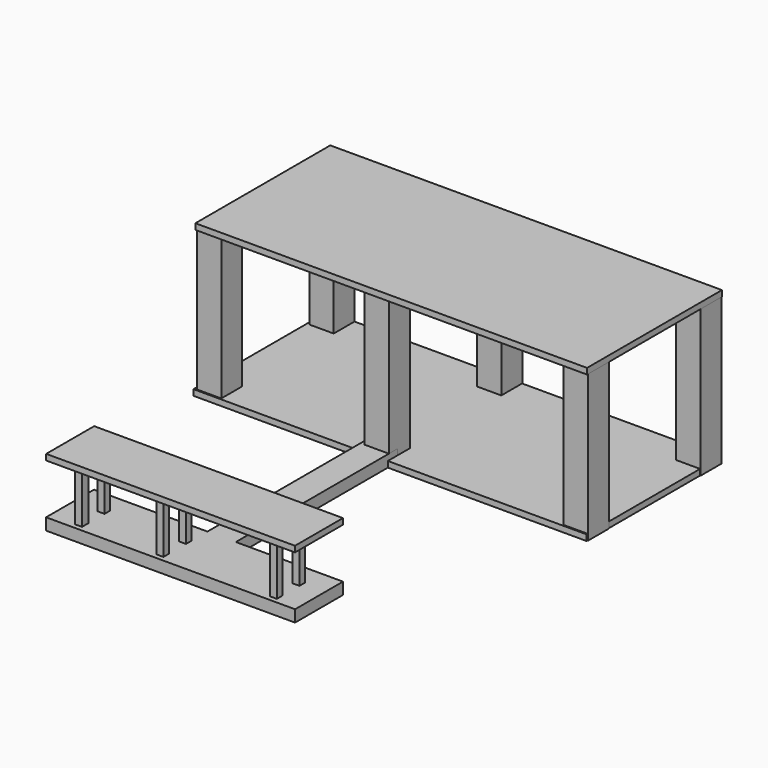
from build123d import *

# Parameters (mm, degrees)
F1_W      = 2.1082
F1_H      = 2.2606
F2_DEPTH  = 12.7
F0_W      = 2.4492868688
F0_H      = 17.4416182563
F3_DEPTH  = 1.016
F4_W      = 0.6096
F4_H      = 0.6012953818
F4_H_2    = 0.7112
F4_H_3    = 0.6096
F5_DEPTH  = 4.318
F6_W      = 21.482726559
F6_H      = 5.1775947213
F6_W_2    = 0.6096
F6_H_2    = 0.6012953818
F7_DEPTH  = 0.508
F8_W      = 33.9498203248
F8_H      = 14.4916079007
F9_DEPTH  = 0.508
F10_W     = 2.1082
F10_H     = 2.2606
F11_DEPTH = 0.508


# Not quite as in the source:
# - a feature names something its author has since deleted; it is built from what else it names


with BuildPart() as f2:
    # F1 (on Top) → F2 (new body)
    with BuildSketch(Plane.XY):
        with Locations((-15.5251261375, 6.3823008758)):
            Rectangle(F1_W, F1_H)
    extrude(amount=F2_DEPTH)


with BuildPart() as f2b:
    # F1 (on Top) → F2, piece 2 (new body)
    with BuildSketch(Plane.XY):
        with Locations((-15.5251261375, -5.7539824548)):
            Rectangle(F1_W, F1_H)
    extrude(amount=F2_DEPTH)


with BuildPart() as f2c:
    # F1 (on Top) → F2, piece 3 (new body)
    with BuildSketch(Plane.XY):
        with Locations((-1.0541, 6.3823008758)):
            Rectangle(F1_W, F1_H)
    extrude(amount=F2_DEPTH)


with BuildPart() as f2d:
    # F1 (on Top) → F2, piece 4 (new body)
    with BuildSketch(Plane.XY):
        with Locations((-1.0541, -5.7539824548)):
            Rectangle(F1_W, F1_H)
    extrude(amount=F2_DEPTH)


with BuildPart() as f2e:
    # F1 (on Top) → F2, piece 5 (new body)
    with BuildSketch(Plane.XY):
        with Locations((16.14880772, 6.3823008758)):
            Rectangle(F1_W, F1_H)
    extrude(amount=F2_DEPTH)


with BuildPart() as f2f:
    # F1 (on Top) → F2, piece 6 (new body)
    with BuildSketch(Plane.XY):
        with Locations((16.14880772, -5.7539824548)):
            Rectangle(F1_W, F1_H)
    extrude(amount=F2_DEPTH)


with BuildPart() as f3:
    # F0 (on Top) → F3 (new body)
    with BuildSketch(Plane.XY):
        with Locations((-1.2246434344, -14.6834761836)):
            Rectangle(F0_W, F0_H)
        Polygon((9.2528564855, -23.4042853117), (0, -23.4042853117), (-2.4492868688, -23.4042853117), (-12.2464280576, -23.4042853117), (-12.2464280576, -28.5750012845), (9.2528564855, -28.5750012845), align=None)
    extrude(amount=F3_DEPTH)

    # F4 (on face) → F5 (join)
    with BuildSketch(Plane.XY.offset(1.016)):
        with Locations((-9.7829406224, -25.4231281579)):
            Rectangle(F4_W, F4_H)
        with Locations((-9.7829406224, -27.8016733074)):
            Rectangle(F4_W, F4_H_2)
        with Locations((-2.7540868688, -25.4231281579)):
            Rectangle(F4_W, F4_H)
        with Locations((-2.7540868688, -27.8524733074)):
            Rectangle(F4_W, F4_H_3)
        with Locations((7.0400689803, -25.4231281579)):
            Rectangle(F4_W, F4_H)
        with Locations((7.0400689803, -27.8524733074)):
            Rectangle(F4_W, F4_H_3)
    extrude(amount=F5_DEPTH)


with BuildPart() as f7:
    # F6 (on face) → F7 (new body)
    with BuildSketch(Plane.XY.offset(5.334)):
        with Locations((-1.4948770404, -25.9876903147)):
            Rectangle(F6_W, F6_H)
        with Locations((-9.7829406224, -25.4231281579)):
            Rectangle(F6_W_2, F6_H_2, mode=Mode.SUBTRACT)
        with Locations((-9.7829406224, -25.4231281579)):
            Rectangle(F6_W_2, F6_H_2)
    extrude(amount=F7_DEPTH)


with BuildPart() as f9:
    # F8 (on Top) → F9 (new body)
    with BuildSketch(Plane.XY):
        with Locations((0.1881280914, 0.2499890979)):
            Rectangle(F8_W, F8_H)
    extrude(amount=F9_DEPTH)


with BuildPart() as f11:
    # F10 (on face) → F11 (new body)
    with BuildSketch(Plane.XY.offset(12.7)):
        Polygon((17.2401238233, 7.5126008758), (-14.4710261375, 7.5126008758), (-14.4710261375, 5.2520008758), (-16.5792261375, 5.2520008758), (-16.5792261375, -7.0438468829), (17.2401238233, -7.0438468829), align=None)
        with Locations((-15.5251261375, 6.3823008758)):
            Rectangle(F10_W, F10_H)
    extrude(amount=F11_DEPTH)


solid = Compound([f2.part, f2b.part, f2c.part, f2d.part, f2e.part, f2f.part, f3.part, f7.part, f9.part, f11.part])
